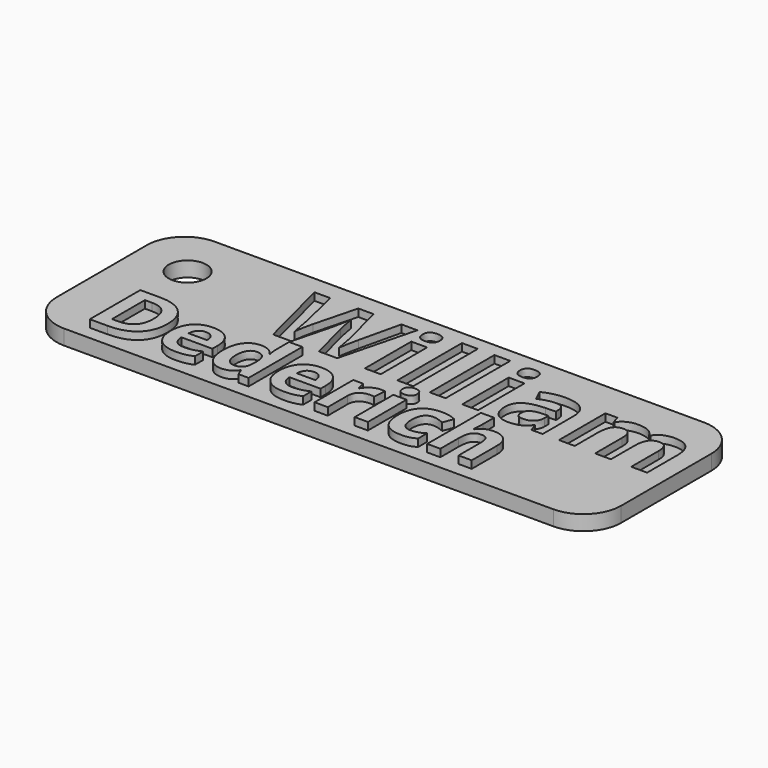
from build123d import *

# Parameters (mm, degrees)
F1_DEPTH     = 2
F3_D         = 5
F4_TEXT_SIZE = 14.1306637993
F5_DEPTH     = 1
F6_TEXT_SIZE = 11.744966226
F7_DEPTH     = 1


# Not quite as in the source:
# - Text() gives the source's letters only with a copy of the font that has no kerning and outlines rounded to 1/6400 em; it was checked with that copy


with BuildPart() as f1:
    # F0 (on Top) → F1 (new body)
    with BuildSketch(Plane.XY):
        with BuildLine():
            Line((32.5, 12.5), (-32.5, 12.5))
            ThreePointArc((-32.5, 12.5), (-36.0355339059, 11.0355339059), (-37.5, 7.5))
            Line((-37.5, 7.5), (-37.5, -7.5))
            ThreePointArc((-37.5, -7.5), (-36.0355339059, -11.0355339059), (-32.5, -12.5))
            Line((-32.5, -12.5), (32.5, -12.5))
            ThreePointArc((32.5, -12.5), (36.0355339059, -11.0355339059), (37.5, -7.5))
            Line((37.5, -7.5), (37.5, 7.5))
            ThreePointArc((37.5, 7.5), (36.0355339059, 11.0355339059), (32.5, 12.5))
        make_face()
    extrude(amount=F1_DEPTH)

    # F3 (through all)
    with Locations(Plane.XY.offset(2)):
        with Locations((-30.5, 5.5)):
            Hole(F3_D / 2)

    # F4 (on face) → F5 (cut)
    with BuildSketch(Plane.XY.offset(2)):
        with Locations((-17.3091460019, 0)):
            Text('William', F4_TEXT_SIZE, font='Open Sans', font_style=FontStyle.BOLD, text_align=(TextAlign.LEFT, TextAlign.BOTTOM))
    extrude(amount=-F5_DEPTH, mode=Mode.SUBTRACT)

    # F6 (on face) → F7 (join)
    with BuildSketch(Plane.XY.offset(2)):
        with Locations((-31.5792784095, -10.7026007026)):
            Text('Dederich', F6_TEXT_SIZE, font='Open Sans', font_style=FontStyle.BOLD, text_align=(TextAlign.LEFT, TextAlign.BOTTOM))
    extrude(amount=F7_DEPTH)


solid = f1.part
